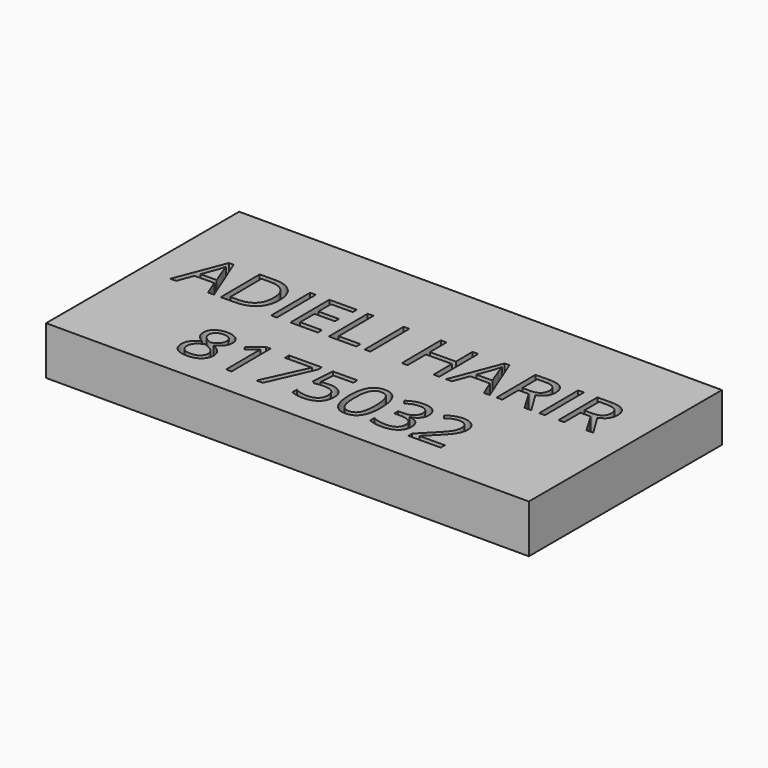
from build123d import *

# Parameters (mm, degrees)
F0_W         = 100
F0_H         = 50
F1_DEPTH     = 10
F2_TEXT_SIZE = 14.2304712411
F3_DEPTH     = 36.8


# Not quite as in the source:
# - Text() gives the source's letters only with a copy of the font that has no kerning and outlines rounded to 1/6400 em; it was checked with that copy


with BuildPart() as f1:
    # F0 (on Top) → F1 (new body)
    with BuildSketch(Plane.XY):
        Rectangle(F0_W, F0_H)
    extrude(amount=F1_DEPTH)

    # F2 (on face) → F3 (cut)
    with BuildSketch(Plane.XY.offset(10)):
        with Locations(Location((-44.0266884015, -0.3048647062), (0, 0, 0.3967407599))):
            Text('ADIELI HARIR', F2_TEXT_SIZE, font='Open Sans', text_align=(TextAlign.LEFT, TextAlign.BOTTOM))
        with Locations(Location((-29.1022364218, -19.5554245679), (0, 0, 0.3967407599))):
            Text('8175032', F2_TEXT_SIZE, font='Open Sans', text_align=(TextAlign.LEFT, TextAlign.BOTTOM))
    extrude(amount=-F3_DEPTH, mode=Mode.SUBTRACT)


solid = f1.part
